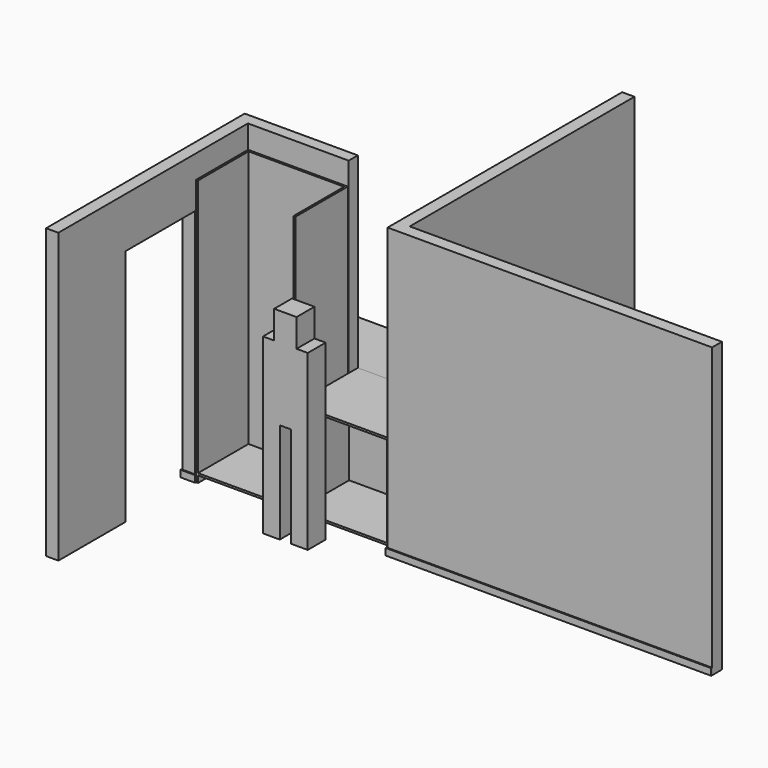
from build123d import *

# Parameters (mm, degrees)
F7_W           = 110
F7_H           = 2580
F8_DEPTH       = 592
F9_W           = 102
F9_H           = 2580
F10_DEPTH      = 1745
F10_DEPTH_BACK = 110
F11_W          = 844
F11_H          = 1690
F12_DEPTH      = 102.001
F13_W          = 110
F13_H          = 2580
F14_DEPTH      = 620
F14_DEPTH_BACK = 2000
F15_W          = 400
F15_H          = 200
F16_DEPTH      = 1550
F17_W          = 100
F17_H          = 200
F18_DEPTH      = 900
F19_W          = 200
F19_H          = 200
F20_DEPTH      = 250
F21_W          = 110
F21_H          = 450
F22_DEPTH      = 775
F23_W          = 110
F23_H          = 2580
F24_DEPTH      = 750
F25_W          = 2790
F25_H          = 2580
F26_DEPTH      = 110
F28_W          = 10
F28_H          = 60
F30_W          = 582
F30_H          = 2380
F31_DEPTH      = 18
F32_W          = 873
F32_H          = 2380
F33_DEPTH      = 18
F34_W          = 18
F34_H          = 2380
F35_DEPTH      = 564
F36_W          = 855
F36_H          = 18
F37_DEPTH      = 564
F38_W          = 834
F38_H          = 890
F39_DEPTH      = 18
F40_W          = 18
F40_H          = 890
F41_DEPTH      = 574
F42_W          = 844
F42_H          = 694
F43_DEPTH      = 18
F44_W          = 798
F44_H          = 18
F45_DEPTH      = 574
F46_W          = 100
F46_H          = 708
F47_DEPTH      = 600


with BuildPart() as f8:
    # F7 (on Front) → F8 (new body)
    with BuildSketch(Plane.XZ):
        with Locations((-55, 1290)):
            Rectangle(F7_W, F7_H)
    extrude(amount=F8_DEPTH)

    # F9 (on face) → F10 (join, two sides)
    with BuildSketch(Plane.YZ) as f10_sk:
        with Locations((51, 1290)):
            Rectangle(F9_W, F9_H)
    extrude(amount=F10_DEPTH)
    extrude(f10_sk.sketch, amount=-F10_DEPTH_BACK)

    # F11 (on face) → F12 (cut, through all)
    with BuildSketch(Plane.XZ):
        with Locations((1323, 1735)):
            Rectangle(F11_W, F11_H)
    extrude(amount=-F12_DEPTH, mode=Mode.SUBTRACT)

    # F13 (on face) → F14 (join, two sides)
    with BuildSketch(Plane.XZ) as f14_sk:
        with Locations((1800, 1290)):
            Rectangle(F13_W, F13_H)
    extrude(amount=F14_DEPTH)
    extrude(f14_sk.sketch, amount=-F14_DEPTH_BACK)

    # F21 (on face) → F22 (join)
    with BuildSketch(Plane.XZ.offset(592)):
        with Locations((-55, 2355)):
            Rectangle(F21_W, F21_H)
    extrude(amount=F22_DEPTH)

    # F23 (on face) → F24 (join)
    with BuildSketch(Plane.XZ.offset(1367)):
        with Locations((-55, 1290)):
            Rectangle(F23_W, F23_H)
    extrude(amount=F24_DEPTH)

    # F25 (on face) → F26 (join)
    with BuildSketch(Plane.XZ.offset(620)):
        with Locations((3250, 1290)):
            Rectangle(F25_W, F25_H)
    extrude(amount=-F26_DEPTH)


with BuildPart() as f16:
    # F15 (on Top) → F16 (new body)
    with BuildSketch(Plane.XY):
        with Locations((1057.8335940038, -803.4160733223)):
            Rectangle(F15_W, F15_H)
    extrude(amount=F16_DEPTH)

    # F17 (on face) → F18 (cut)
    with BuildSketch(Plane(origin=(0, 0, 0), x_dir=(1, 0, 0), z_dir=(0, 0, -1))):
        with Locations((1057.8335940038, 803.4160733223)):
            Rectangle(F17_W, F17_H)
    extrude(amount=-F18_DEPTH, mode=Mode.SUBTRACT)

    # F19 (on face) → F20 (join)
    with BuildSketch(Plane.XY.offset(1550)):
        with Locations((1057.8335940038, -803.4160733223)):
            Rectangle(F19_W, F19_H)
    extrude(amount=F20_DEPTH)


with BuildPart() as f29:
    # F29: sweep along a path in F29_path
    with BuildLine(Plane(origin=(0, -592, 0), x_dir=(0, 1, 0), z_dir=(0, 0, 1))) as f29_path:
        Line((-28, -4645), (-28, -1745))
        Line((-28, -1745), (592, -1745))
        Line((592, -1745), (592, 0))
        Line((592, 0), (0, 0))
        Line((0, 0), (0, 110))
        Line((0, 110), (694, 110))
        Line((694, 110), (694, -1745))
        Line((694, -1745), (2592, -1745))
    # F28 (on face) → F29 (sweep)
    with BuildSketch(Plane.XZ.offset(592)):
        with Locations((5, 30)):
            Rectangle(F28_W, F28_H)
    sweep(path=f29_path.line, transition=Transition.RIGHT)


with BuildPart() as f31:
    # F30 (on face) → F31 (new body)
    with BuildSketch(Plane.YZ.offset(10)):
        with Locations((-301, 1190)):
            Rectangle(F30_W, F30_H)
    extrude(amount=F31_DEPTH)

    # F32 (on face) → F33 (join)
    with BuildSketch(Plane.XZ.offset(10)):
        with Locations((464.5, 1190)):
            Rectangle(F32_W, F32_H)
    extrude(amount=F33_DEPTH)

    # F34 (on face) → F35 (join, through all)
    with BuildSketch(Plane.XZ.offset(28)):
        with Locations((892, 1190)):
            Rectangle(F34_W, F34_H)
    extrude(amount=F35_DEPTH)

    # F36 (on face) → F37 (join, through all)
    with BuildSketch(Plane.XZ.offset(28)):
        with Locations((455.5, 69)):
            Rectangle(F36_W, F36_H)
    extrude(amount=F37_DEPTH)


with BuildPart() as f39:
    # F38 (on face) → F39 (new body)
    with BuildSketch(Plane.XZ):
        with Locations((1318, 445)):
            Rectangle(F38_W, F38_H)
    extrude(amount=F39_DEPTH)

    # F40 (on face) → F41 (join, through all)
    with BuildSketch(Plane.XZ.offset(18)):
        with Locations((910, 445)):
            Rectangle(F40_W, F40_H)
        with Locations((1726, 445)):
            Rectangle(F40_W, F40_H)
    extrude(amount=F41_DEPTH)

    # F42 (on face) → F43 (join)
    with BuildSketch(Plane.XY.offset(890)):
        with Locations((1323, -245)):
            Rectangle(F42_W, F42_H)
    extrude(amount=F43_DEPTH)

    # F44 (on face) → F45 (join, through all)
    with BuildSketch(Plane.XZ.offset(18)):
        with Locations((1318, 69)):
            Rectangle(F44_W, F44_H)
    extrude(amount=F45_DEPTH)


with BuildPart() as f47:
    # F46 (on face) → F47 (new body)
    with BuildSketch(Plane(origin=(0, 102, 0), x_dir=(-1, 0, 0), z_dir=(0, 1, 0))):
        Polygon((110, 908), (-1745, 908), (-1745, 808), (-1645, 808), (10, 808), (110, 808), align=None)
        with Locations((-1695, 454)):
            Rectangle(F46_W, F46_H)
        with Locations((60, 454)):
            Rectangle(F46_W, F46_H)
    extrude(amount=F47_DEPTH)


solid = Compound([f8.part, f16.part, f29.part, f31.part, f39.part, f47.part])
